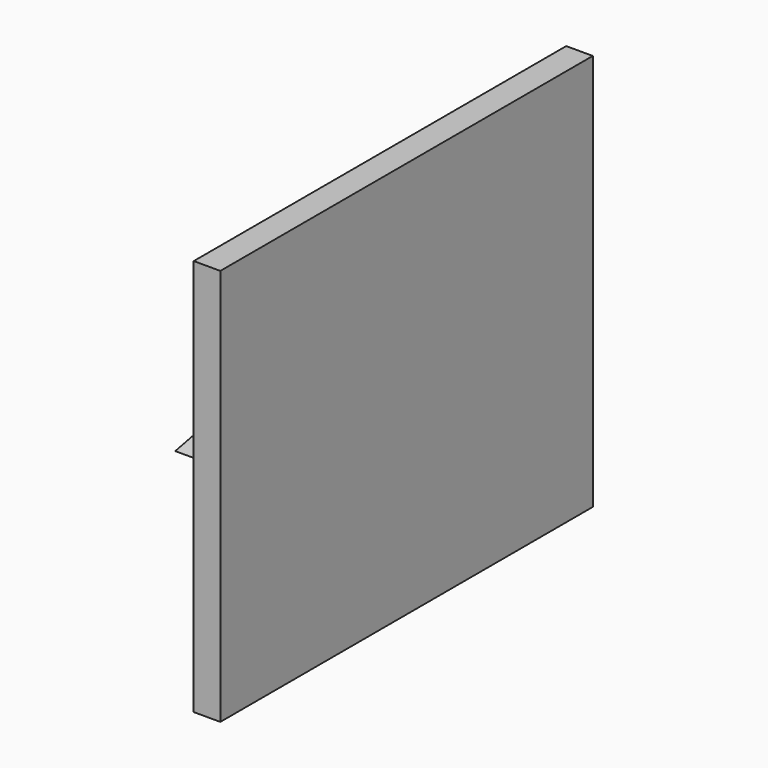
from build123d import *

# Parameters (mm, degrees)
F1_DEPTH = 5.08
F2_W     = 53.3400028944
F2_H     = 45.4899612814
F3_DEPTH = 3.048
F4_W     = 3.1429869445
F4_H     = 15.7159869445
F4_W_2   = 6.2865
F4_H_2   = 5.2390130555
F5_DEPTH = 5.08


with BuildPart() as f1:
    # F0 (on Right) → F1 (new body)
    with BuildSketch(Plane.YZ):
        Polygon((12.7, 7.9436706283), (-12.7, 7.9436706283), (-12.7, -2.7003783846), (-12.6387012167, -2.5758128428), (-12.4020947161, -2.2278213751), (-11.9941407446, -1.7776895645), (-11.4932424625, -1.3618151002), (-11.0641874235, -1.077066095), (-10.9145848638, -0.9940952884), (-10.7109237259, -0.8800256144), (-9.5911579813, -0.4484073484), (-8.5116021006, -0.2446854706), (-8.1517541896, -0.2446854706), (-7.7411519552, -0.2446854706), (-6.5080332683, -0.4957845293), (-5.3203845271, -1.0414724693), (-5.1114511593, -1.1891920898), (-4.9565763698, -1.297916646), (-4.5242292241, -1.6715768273), (-4.0193828436, -2.2298136463), (-3.6048082147, -2.8526413552), (-3.3530653122, -3.3535274892), (-3.2864821511, -3.5275232231), (-3.2199232859, -3.3482552594), (-2.9450870447, -2.8394486325), (-2.4652776821, -2.208056587), (-1.8668552954, -1.6438915465), (-1.3488283402, -1.2675466582), (-1.1656001301, -1.1594295018), (-0.9171371863, -1.0118313613), (0.4675763315, -0.4734322183), (1.9781795225, -0.2394618327), (2.2898970768, -0.2446854706), (2.6048945898, -0.2479654292), (3.5507374885, -0.3553537059), (4.7101421411, -0.6658564608), (5.7467305632, -1.1857906512), (6.4413529232, -1.7177149127), (6.6411874426, -1.9259801407), (6.848675199, -2.1434656971), (7.3714034282, -2.8948191942), (7.9183061677, -4.1042006986), (8.2617299893, -5.5640495661), (8.3810233012, -6.8545067898), (8.3810233012, -7.2848859603), (8.3810233012, -13.7391643503), (12.7, -13.7391643503), align=None)
    extrude(amount=-F1_DEPTH)


with BuildPart() as f1b:
    # F0 (on Right) → F1, piece 2 (new body)
    with BuildSketch(Plane.YZ):
        Polygon((-5.0270954813, -13.7391643503), (-5.0270954813, -6.7708071036), (-5.0270954813, -6.3799818051), (-5.3019195745, -5.2074937618), (-5.9023342325, -4.1417744475), (-6.0651416628, -3.9677665656), (-6.18640295, -3.8379409419), (-6.602933406, -3.4991819505), (-7.2297092133, -3.1498784993), (-7.9342564853, -2.9304006718), (-8.512926232, -2.8552653221), (-8.7053626224, -2.8552653221), (-9.0704949112, -2.8552653221), (-10.1638873584, -3.1327376782), (-11.2566359619, -3.7292042378), (-11.4444682622, -3.8886952655), (-11.5835385101, -4.0060084542), (-11.9578911272, -4.4093461876), (-12.3539886555, -5.0071368786), (-12.6097039524, -5.6675261883), (-12.7, -6.1980777265), (-12.7, -6.375365567), (-12.7, -13.7391643503), align=None)
    extrude(amount=-F1_DEPTH)


with BuildPart() as f1c:
    # F0 (on Right) → F1, piece 3 (new body)
    with BuildSketch(Plane.YZ):
        Polygon((2.1224977043, -2.8552653221), (1.9339608203, -2.8552653221), (1.5438886976, -2.8552653221), (0.3733078895, -3.165683041), (-0.7497256657, -3.8300325971), (-0.9382261058, -4.0073204377), (-1.1273825375, -4.1839522864), (-1.8424621212, -5.2411072643), (-2.1792409894, -6.3582247459), (-2.1792409894, -6.7312532315), (-2.1792409894, -13.7391643503), (5.5331688093, -13.7391643503), (5.5331688093, -7.3639694084), (5.5331688093, -7.0766085843), (5.4639252372, -6.2158745393), (5.2655484772, -5.2575799456), (4.9466636058, -4.4772413322), (4.6428422482, -4.001404364), (4.5196615779, -3.8636339516), (4.4042556244, -3.7344643197), (3.99365339, -3.4055937962), (3.3800581573, -3.0925278145), (2.6899305556, -2.912603859), align=None)
    extrude(amount=-F1_DEPTH)


with BuildPart() as f3:
    # F2 (on Right) → F3 (new body)
    with BuildSketch(Plane.YZ):
        with Locations((0.1006424427, 0.1006415114)):
            Rectangle(F2_W, F2_H)
    extrude(amount=F3_DEPTH)

    # F4 (on Right) → F5 (join)
    with BuildSketch(Plane.YZ):
        Polygon((22.8713592142, -4.7150065277), (18.3754403267, -4.7150065277), (18.3754403267, 0.5345287472), (21.5106859241, 0.5345287472), (22.5582480273, 3.6669934723), (18.3754403267, 3.6669934723), (18.3754403267, 7.8501769664), (15.2323782235, 7.8501769664), (15.2323782235, -5.7624934723), (15.2323782235, -5.9916523798), (15.363229538, -6.6791291023), (15.755933799, -7.3339869445), (16.4104910064, -7.7266912055), (17.0979677289, -7.8579934723), (17.32750243, -7.8579934723), (22.8713592142, -7.8579934723), align=None)
        with Locations((12.0192682024, 0)):
            Rectangle(F4_W, F4_H)
        Polygon((6.9401177235, 3.6669934723), (6.7110339747, 3.6669934723), (-1.6709660253, 3.6669934723), (-1.9005007263, 3.6669934723), (-2.5879774488, 3.536066999), (-3.2429104498, 3.1434378968), (-3.6356147107, 2.4885800545), (-3.7663908665, 1.8010281733), (-3.7663908665, 1.5714934723), (-3.7663908665, -5.7624934723), (-3.7663908665, -5.9916523798), (-3.6356147107, -6.6791291023), (-3.2429104498, -7.3339869445), (-2.5879774488, -7.7266912055), (-1.9005007263, -7.8579934723), (-1.6709660253, -7.8579934723), (6.7110339747, -7.8579934723), (6.9401177235, -7.8579934723), (7.6276696047, -7.7266912055), (8.2820764947, -7.3339869445), (8.6747807557, -6.6791291023), (8.8060830225, -5.9916523798), (8.8060830225, -5.7624934723), (8.8060830225, 1.5714934723), (8.8060830225, 1.8010281733), (8.6747807557, 2.4885800545), (8.2820764947, 3.1434378968), (7.6276696047, 3.536066999), align=None)
        with Locations((2.519846078, -2.0955)):
            Rectangle(F4_W_2, F4_H_2, mode=Mode.SUBTRACT)
        Polygon((-17.9749947186, 2.5244307593), (-14.8371937251, 3.1715472544), (-14.8371937251, 7.8579934723), (-17.9806316219, 7.8579934723), align=None)
        Polygon((-7.2740478731, 3.6669934723), (-7.5031316219, 3.6669934723), (-22.8713592142, 0.5240065277), (-8.5506937251, 0.5240065277), (-8.5506937251, -4.7150065277), (-14.8371937251, -4.7150065277), (-14.8371937251, -0.4689151931), (-17.9806316219, -0.4689151931), (-17.9806316219, -5.7624934723), (-17.9806316219, -5.9916523798), (-17.8497803074, -6.6791291023), (-17.4570760464, -7.3339869445), (-16.8021430454, -7.7266912055), (-16.1146663229, -7.8579934723), (-15.8851316219, -7.8579934723), (-7.5031316219, -7.8579934723), (-7.2740478731, -7.8579934723), (-6.5865711506, -7.7266912055), (-5.9317133083, -7.3339869445), (-5.5390090474, -6.6791291023), (-5.4077067806, -5.9916523798), (-5.4077067806, -5.7624934723), (-5.4077067806, 1.5714934723), (-5.4077067806, 1.8010281733), (-5.5390090474, 2.4885800545), (-5.9317133083, 3.1434378968), (-6.5865711506, 3.536066999), align=None)
    extrude(amount=-F5_DEPTH)


solid = Compound([f1.part, f1b.part, f1c.part, f3.part])
